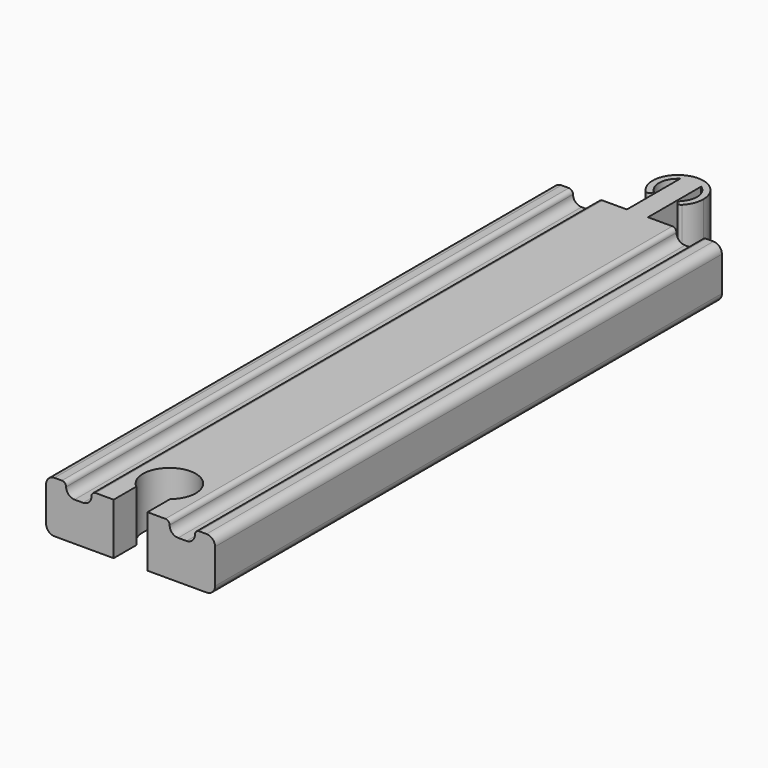
from build123d import *

# Parameters (mm, degrees)
F1_DEPTH = 150
F2_R     = 1.99999
F4_DEPTH = 12.2
F5_DEPTH = 25


# Not quite as in the source:
# - a fillet or chamfer is up to 0.001 mm smaller than in the source, because OpenCascade refuses the exact size


with BuildPart() as f1:
    # F0 (on Front) → F1 (new body)
    with BuildSketch(Plane.XZ):
        with BuildLine():
            ThreePointArc((20, 4.1), (19.4142135624, 5.5142135624), (18, 6.1))
            Line((18, 6.1), (16.25, 6.1))
            ThreePointArc((16.25, 6.1), (15.5428932188, 5.8071067812), (15.25, 5.1))
            Line((15.25, 5.1), (15.25, 3.1))
            Line((15.25, 3.1), (9.25, 3.1))
            Line((9.25, 3.1), (9.25, 5.1))
            ThreePointArc((9.25, 5.1), (8.9571067812, 5.8071067812), (8.25, 6.1))
            Line((8.25, 6.1), (-8.25, 6.1))
            ThreePointArc((-8.25, 6.1), (-8.9571067812, 5.8071067812), (-9.25, 5.1))
            Line((-9.25, 5.1), (-9.25, 3.1))
            Line((-9.25, 3.1), (-15.25, 3.1))
            Line((-15.25, 3.1), (-15.25, 5.1))
            ThreePointArc((-15.25, 5.1), (-15.5428932188, 5.8071067812), (-16.25, 6.1))
            Line((-16.25, 6.1), (-18, 6.1))
            ThreePointArc((-18, 6.1), (-19.4142135624, 5.5142135624), (-20, 4.1))
            Line((-20, 4.1), (-20, -4.1))
            ThreePointArc((-20, -4.1), (-19.4142135624, -5.5142135624), (-18, -6.1))
            Line((-18, -6.1), (18, -6.1))
            ThreePointArc((18, -6.1), (19.4142135624, -5.5142135624), (20, -4.1))
            Line((20, -4.1), (20, 4.1))
        make_face()
    extrude(amount=F1_DEPTH)

    # F2 (radius 2 in the source; OpenCascade refuses exactly that, so slightly less here)
    f2_edges = [f1.edges().sort_by_distance(p)[0] for p in [
        (15.25, -75, 3.1),
        (9.25, -75, 3.1),
        (-9.25, -75, 3.1),
        (-15.25, -75, 3.1),
    ]]
    fillet(f2_edges, radius=F2_R)

    # F3 (on face) → F4 (join)
    with BuildSketch(Plane(origin=(0, 0, -6.1), x_dir=(1, 0, 0), z_dir=(0, 0, -1))):
        with BuildLine():
            Line((0, 0), (-2.5, 0))
            Line((-2.5, 0), (-2.5, -6.5456439427))
            ThreePointArc((-2.5, -6.5456439427), (-1.2794263668, -6.1379979383), (0, -6))
            Line((0, -6), (0, 0))
        make_face()
        with BuildLine():
            Line((2.5, -6.5456439427), (2.5, 0))
            Line((2.5, 0), (0, 0))
            Line((0, 0), (0, -6))
            ThreePointArc((0, -6), (1.2794263668, -6.1379979383), (2.5, -6.5456439427))
        make_face()
        with BuildLine():
            Line((2.5, -8.2583426132), (2.5, -6.5456439427))
            ThreePointArc((2.5, -6.5456439427), (1.2794263668, -6.1379979383), (0, -6))
            Line((0, -6), (0, -7.5))
            ThreePointArc((0, -7.5), (1.3062430401, -7.6937569599), (2.5, -8.2583426132))
        make_face()
        with BuildLine():
            ThreePointArc((0, -6), (-1.2794263668, -6.1379979383), (-2.5, -6.5456439427))
            Line((-2.5, -6.5456439427), (-2.5, -8.2583426132))
            ThreePointArc((-2.5, -8.2583426132), (-1.3062430401, -7.6937569599), (0, -7.5))
            Line((0, -7.5), (0, -6))
        make_face()
        with BuildLine():
            Line((2.5, -15.7416573868), (2.5, -8.2583426132))
            ThreePointArc((2.5, -8.2583426132), (1.3062430401, -7.6937569599), (0, -7.5))
            ThreePointArc((0, -7.5), (-1.3062430401, -7.6937569599), (-2.5, -8.2583426132))
            Line((-2.5, -8.2583426132), (-2.5, -15.7416573868))
            ThreePointArc((-2.5, -15.7416573868), (0, -16.5), (2.5, -15.7416573868))
        make_face()
        with BuildLine():
            ThreePointArc((6, -12), (5.5549205986, -9.7322131619), (4.2857142857, -7.8008747267))
            ThreePointArc((4.2857142857, -7.8008747267), (3.2251093408, -7.7900511001), (3.2142857143, -8.850656045))
            ThreePointArc((3.2142857143, -8.850656045), (4.166190449, -10.2991598715), (4.5, -12))
            ThreePointArc((4.5, -12), (3.9686269666, -14.1213203436), (2.5, -15.7416573868))
            ThreePointArc((2.5, -15.7416573868), (0, -16.5), (-2.5, -15.7416573868))
            ThreePointArc((-2.5, -15.7416573868), (-4.4760183399, -12.4639610121), (-3.2142857143, -8.850656045))
            ThreePointArc((-3.2142857143, -8.850656045), (-3.2251093408, -7.7900511001), (-4.2857142857, -7.8008747267))
            ThreePointArc((-4.2857142857, -7.8008747267), (-2.2677868381, -17.5549205986), (6, -12))
        make_face()
    extrude(amount=-F4_DEPTH)

    # F3 (on face) → F5 (cut)
    with BuildSketch(Plane(origin=(0, 0, -6.1), x_dir=(1, 0, 0), z_dir=(0, 0, -1))):
        with BuildLine():
            ThreePointArc((-4, 143.3023431781), (0, 144.75), (4, 143.3023431781))
            Line((4, 143.3023431781), (4, 150))
            Line((4, 150), (-4, 150))
            Line((-4, 150), (-4, 143.3023431781))
        make_face()
        with BuildLine():
            ThreePointArc((-4, 143.3023431781), (-2.6516504294, 132.8403842887), (6.25, 138.5))
            ThreePointArc((6.25, 138.5), (5.6596157113, 141.1516504294), (4, 143.3023431781))
            ThreePointArc((4, 143.3023431781), (0, 144.75), (-4, 143.3023431781))
        make_face()
    extrude(amount=-F5_DEPTH, mode=Mode.SUBTRACT)


solid = f1.part
